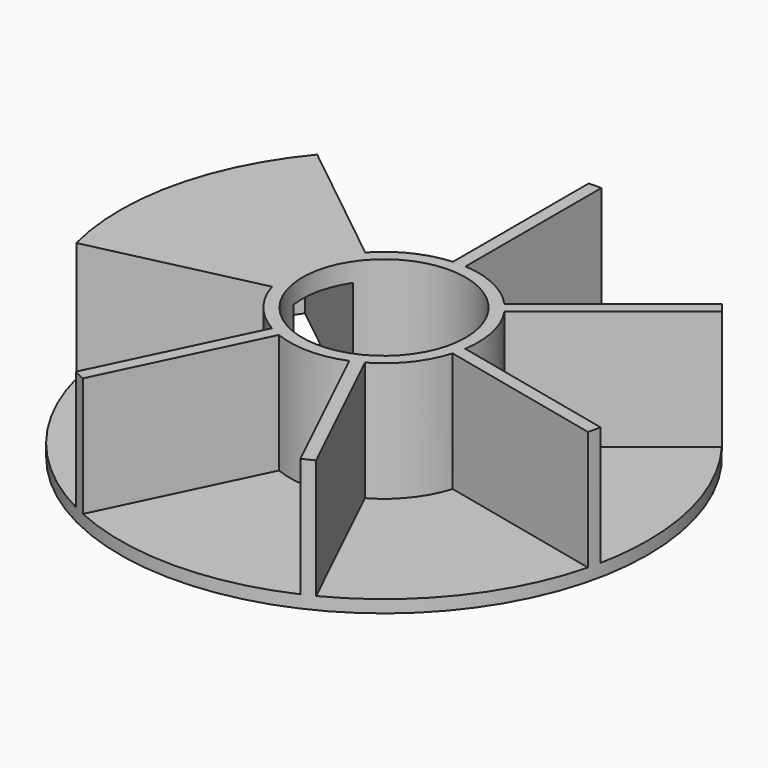
from build123d import *

# Parameters (mm, degrees)
F0_R     = 42
F0_R_2   = 13
F3_DEPTH = 21
F4_DEPTH = 25
F9_DEPTH = 18


# Not quite as in the source:
# - a feature names something its author has since deleted; it is built from what else it names


with BuildPart() as f3:
    # F0 (on Top) → F3 (new body)
    with BuildSketch(Plane.XY):
        Circle(F0_R)
        Circle(F0_R_2, mode=Mode.SUBTRACT)
    extrude(amount=F3_DEPTH)

    # F2 (on offset) → F4 (cut)
    with BuildSketch(Plane.XY.offset(2)):
        with BuildLine():
            Line((1, 43.9886348958), (1, 14.9666295471))
            ThreePointArc((1, 14.9666295471), (6.5082560868, 13.5145330185), (11.0778923645, 10.1133723733))
            Line((11.0778923645, 10.1133723733), (33.7682098305, 28.2082967377))
            ThreePointArc((33.7682098305, 28.2082967377), (19.0908845212, 39.6426301877), (1, 43.9886348958))
        make_face()
        with BuildLine():
            ThreePointArc((-11.0778923645, 10.1133723733), (-6.5082560868, 13.5145330185), (-1, 14.9666295471))
            Line((-1, 14.9666295471), (-1, 43.9886348958))
            ThreePointArc((-1, 43.9886348958), (-19.0908845212, 39.6426301877), (-33.7682098305, 28.2082967377))
            Line((-33.7682098305, 28.2082967377), (-11.0778923645, 10.1133723733))
        make_face()
        with BuildLine():
            ThreePointArc((-7.3947460578, -13.0505835402), (-11.727472237, -9.3523470279), (-14.3688639628, -4.3053162972))
            Line((-14.3688639628, -4.3053162972), (-42.6632270448, -10.7633200327))
            ThreePointArc((-42.6632270448, -10.7633200327), (-34.4005852286, -27.4335512818), (-19.9869222552, -39.1985068436))
            Line((-19.9869222552, -39.1985068436), (-7.3947460578, -13.0505835402))
        make_face()
        with BuildLine():
            ThreePointArc((5.592808322, -13.9183510185), (0, -15), (-5.592808322, -13.9183510185))
            Line((-5.592808322, -13.9183510185), (-18.1849845194, -40.0662743218))
            ThreePointArc((-18.1849845194, -40.0662743218), (0, -44), (18.1849845194, -40.0662743218))
            Line((18.1849845194, -40.0662743218), (5.592808322, -13.9183510185))
        make_face()
        with BuildLine():
            ThreePointArc((14.3688639628, -4.3053162972), (11.727472237, -9.3523470279), (7.3947460578, -13.0505835402))
            Line((7.3947460578, -13.0505835402), (19.9869222552, -39.1985068436))
            ThreePointArc((19.9869222552, -39.1985068436), (34.4005852286, -27.4335512818), (42.6632270448, -10.7633200327))
            Line((42.6632270448, -10.7633200327), (14.3688639628, -4.3053162972))
        make_face()
        with BuildLine():
            ThreePointArc((12.3248719682, 8.5497094083), (14.6239186827, 3.3378140093), (14.8139058307, -2.3554604728))
            Line((14.8139058307, -2.3554604728), (43.1082689127, -8.8134642083))
            ThreePointArc((43.1082689127, -8.8134642083), (42.896828136, 9.7909210941), (35.0151894342, 26.6446337728))
            Line((35.0151894342, 26.6446337728), (12.3248719682, 8.5497094083))
        make_face()
    extrude(amount=F4_DEPTH, mode=Mode.SUBTRACT)

    # F8 (on offset) → F9 (cut)
    with BuildSketch(Plane.XY):
        with BuildLine():
            Line((-39.2080294912, -7.9232600118), (-12.8590309309, -1.9092730337))
            ThreePointArc((-12.8590309309, -1.9092730337), (-12.6740628584, 2.8927721414), (-10.7571840173, 7.2995199854))
            Line((-10.7571840173, 7.2995199854), (-31.8874402635, 24.150337042))
            ThreePointArc((-31.8874402635, 24.150337042), (-38.9976968795, 8.900969829), (-39.2080294912, -7.9232600118))
        make_face()
    extrude(amount=F9_DEPTH, mode=Mode.SUBTRACT)


solid = f3.part
